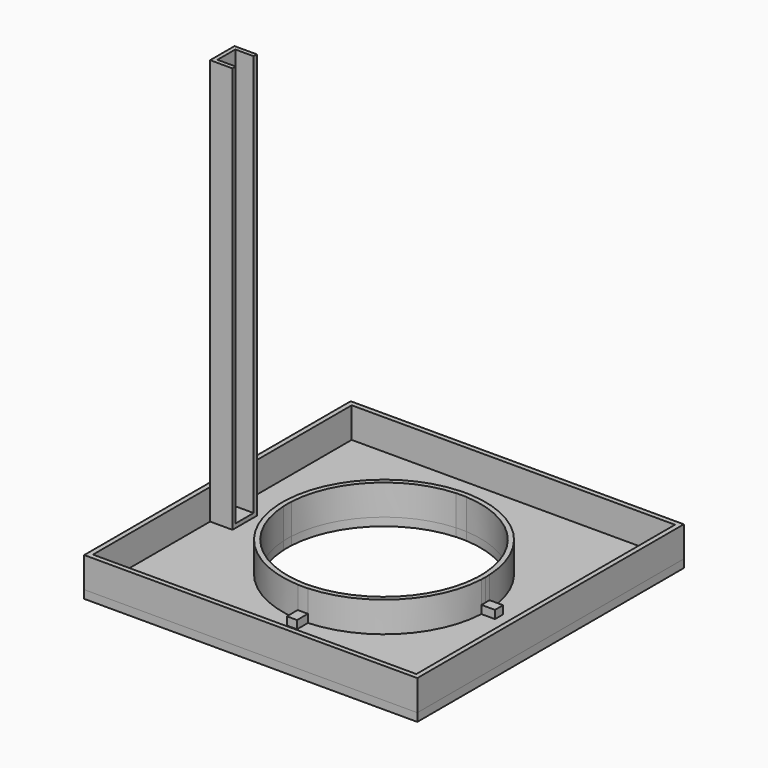
from build123d import *

# Parameters (mm, degrees)
F1_DEPTH = 7.5
F0_W     = 82
F0_H     = 82
F0_R     = 32.8
F0_W_2   = 5.5
F0_H_2   = 7.5
F2_DEPTH = 2
F3_DEPTH = 2
F4_DEPTH = 100
F5_T     = -1


# Not quite as in the source:
# - a feature names something its author has since deleted; it is built from what else it names


with BuildPart() as f1:
    # F0 (on Top) → F1 (new body)
    with BuildSketch(Plane.XY):
        with BuildLine():
            ThreePointArc((-24.9687304443, -1.25), (-17.6776695297, -17.6776695297), (-1.25, -24.9687304443))
            Line((-1.25, -24.9687304443), (-1.25, -23.7671517015))
            ThreePointArc((-1.25, -23.7671517015), (-16.8291413922, -16.8291413922), (-23.7671517015, -1.25))
            Line((-23.7671517015, -1.25), (-24.9687304443, -1.25))
        make_face()
        with BuildLine():
            Line((-1.25, 23.7671517015), (-1.25, 24.9687304443))
            ThreePointArc((-1.25, 24.9687304443), (-17.6776695297, 17.6776695297), (-24.9687304443, 1.25))
            Line((-24.9687304443, 1.25), (-23.7671517015, 1.25))
            ThreePointArc((-23.7671517015, 1.25), (-16.8291413922, 16.8291413922), (-1.25, 23.7671517015))
        make_face()
        with BuildLine():
            Line((23.7671517015, 1.25), (24.9687304443, 1.25))
            ThreePointArc((24.9687304443, 1.25), (17.6776695297, 17.6776695297), (1.25, 24.9687304443))
            Line((1.25, 24.9687304443), (1.25, 23.7671517015))
            ThreePointArc((1.25, 23.7671517015), (16.8291413922, 16.8291413922), (23.7671517015, 1.25))
        make_face()
        with BuildLine():
            ThreePointArc((1.25, -24.9687304443), (17.6776695297, -17.6776695297), (24.9687304443, -1.25))
            Line((24.9687304443, -1.25), (23.7671517015, -1.25))
            ThreePointArc((23.7671517015, -1.25), (16.8291413922, -16.8291413922), (1.25, -23.7671517015))
            Line((1.25, -23.7671517015), (1.25, -24.9687304443))
        make_face()
        with BuildLine():
            Line((1.25, 23.7671517015), (1.25, 24.9687304443))
            ThreePointArc((1.25, 24.9687304443), (0, 25), (-1.25, 24.9687304443))
            Line((-1.25, 24.9687304443), (-1.25, 23.7671517015))
            ThreePointArc((-1.25, 23.7671517015), (0, 23.8), (1.25, 23.7671517015))
        make_face()
        with BuildLine():
            ThreePointArc((-1.25, -24.9687304443), (0, -25), (1.25, -24.9687304443))
            Line((1.25, -24.9687304443), (1.25, -23.7671517015))
            ThreePointArc((1.25, -23.7671517015), (0, -23.8), (-1.25, -23.7671517015))
            Line((-1.25, -23.7671517015), (-1.25, -24.9687304443))
        make_face()
        with BuildLine():
            ThreePointArc((24.9687304443, -1.25), (24.9921813885, -0.6251955264), (25, 0))
            ThreePointArc((25, 0), (24.9921813885, 0.6251955264), (24.9687304443, 1.25))
            Line((24.9687304443, 1.25), (23.7671517015, 1.25))
            ThreePointArc((23.7671517015, 1.25), (23.7917865081, 0.6252157649), (23.8, 0))
            ThreePointArc((23.8, 0), (23.7917865081, -0.6252157649), (23.7671517015, -1.25))
            Line((23.7671517015, -1.25), (24.9687304443, -1.25))
        make_face()
        with BuildLine():
            Line((-23.7671517015, 1.25), (-24.9687304443, 1.25))
            ThreePointArc((-24.9687304443, 1.25), (-25, 0), (-24.9687304443, -1.25))
            Line((-24.9687304443, -1.25), (-23.7671517015, -1.25))
            ThreePointArc((-23.7671517015, -1.25), (-23.8, 0), (-23.7671517015, 1.25))
        make_face()
    extrude(amount=F1_DEPTH)


with BuildPart() as f1b:
    # F0 (on Top) → F1, piece 2 (new body)
    with BuildSketch(Plane.XY):
        Rectangle(F0_W, F0_H)
        Polygon((-39.8, 3.75), (-39.8, 39.8), (39.8, 39.8), (39.8, -39.8), (-39.8, -39.8), (-39.8, -3.75), align=None, mode=Mode.SUBTRACT)
    extrude(amount=F1_DEPTH)


with BuildPart() as f2:
    # F0 (on Top) → F2 (new body)
    with BuildSketch(Plane.XY):
        Rectangle(F0_W, F0_H)
        Polygon((-39.8, 3.75), (-39.8, 39.8), (39.8, 39.8), (39.8, -39.8), (-39.8, -39.8), (-39.8, -3.75), align=None, mode=Mode.SUBTRACT)
        Polygon((39.8, 39.8), (-39.8, 39.8), (-39.8, 3.75), (-34.3, 3.75), (-34.3, -3.75), (-39.8, -3.75), (-39.8, -39.8), (39.8, -39.8), align=None)
        Circle(F0_R, mode=Mode.SUBTRACT)
        Circle(F0_R)
        with BuildLine():
            ThreePointArc((1.25, 24.9687304443), (17.6776695297, 17.6776695297), (24.9687304443, 1.25))
            Line((24.9687304443, 1.25), (28.325, 1.25))
            Line((28.325, 1.25), (28.325, -1.25))
            Line((28.325, -1.25), (24.9687304443, -1.25))
            ThreePointArc((24.9687304443, -1.25), (17.6776695297, -17.6776695297), (1.25, -24.9687304443))
            Line((1.25, -24.9687304443), (1.25, -28.325))
            Line((1.25, -28.325), (-1.25, -28.325))
            Line((-1.25, -28.325), (-1.25, -24.9687304443))
            ThreePointArc((-1.25, -24.9687304443), (-17.6776695297, -17.6776695297), (-24.9687304443, -1.25))
            Line((-24.9687304443, -1.25), (-28.325, -1.25))
            Line((-28.325, -1.25), (-28.325, 1.25))
            Line((-28.325, 1.25), (-24.9687304443, 1.25))
            ThreePointArc((-24.9687304443, 1.25), (-17.6776695297, 17.6776695297), (-1.25, 24.9687304443))
            Line((-1.25, 24.9687304443), (-1.25, 28.325))
            Line((-1.25, 28.325), (1.25, 28.325))
            Line((1.25, 28.325), (1.25, 24.9687304443))
        make_face(mode=Mode.SUBTRACT)
        with BuildLine():
            Line((23.7671517015, 1.25), (24.9687304443, 1.25))
            ThreePointArc((24.9687304443, 1.25), (17.6776695297, 17.6776695297), (1.25, 24.9687304443))
            Line((1.25, 24.9687304443), (1.25, 23.7671517015))
            ThreePointArc((1.25, 23.7671517015), (16.8291413922, 16.8291413922), (23.7671517015, 1.25))
        make_face()
        with BuildLine():
            Line((-1.25, 23.7671517015), (-1.25, 24.9687304443))
            ThreePointArc((-1.25, 24.9687304443), (-17.6776695297, 17.6776695297), (-24.9687304443, 1.25))
            Line((-24.9687304443, 1.25), (-23.7671517015, 1.25))
            ThreePointArc((-23.7671517015, 1.25), (-16.8291413922, 16.8291413922), (-1.25, 23.7671517015))
        make_face()
        with BuildLine():
            ThreePointArc((-24.9687304443, -1.25), (-17.6776695297, -17.6776695297), (-1.25, -24.9687304443))
            Line((-1.25, -24.9687304443), (-1.25, -23.7671517015))
            ThreePointArc((-1.25, -23.7671517015), (-16.8291413922, -16.8291413922), (-23.7671517015, -1.25))
            Line((-23.7671517015, -1.25), (-24.9687304443, -1.25))
        make_face()
        with BuildLine():
            ThreePointArc((1.25, -24.9687304443), (17.6776695297, -17.6776695297), (24.9687304443, -1.25))
            Line((24.9687304443, -1.25), (23.7671517015, -1.25))
            ThreePointArc((23.7671517015, -1.25), (16.8291413922, -16.8291413922), (1.25, -23.7671517015))
            Line((1.25, -23.7671517015), (1.25, -24.9687304443))
        make_face()
        with Locations((-37.05, 0)):
            Rectangle(F0_W_2, F0_H_2)
        with BuildLine():
            ThreePointArc((-24.9687304443, -1.25), (-25, 0), (-24.9687304443, 1.25))
            Line((-24.9687304443, 1.25), (-28.325, 1.25))
            Line((-28.325, 1.25), (-28.325, -1.25))
            Line((-28.325, -1.25), (-24.9687304443, -1.25))
        make_face()
        with BuildLine():
            Line((1.25, -28.325), (1.25, -24.9687304443))
            ThreePointArc((1.25, -24.9687304443), (0, -25), (-1.25, -24.9687304443))
            Line((-1.25, -24.9687304443), (-1.25, -28.325))
            Line((-1.25, -28.325), (1.25, -28.325))
        make_face()
        with BuildLine():
            ThreePointArc((-1.25, 24.9687304443), (0, 25), (1.25, 24.9687304443))
            Line((1.25, 24.9687304443), (1.25, 28.325))
            Line((1.25, 28.325), (-1.25, 28.325))
            Line((-1.25, 28.325), (-1.25, 24.9687304443))
        make_face()
        with BuildLine():
            ThreePointArc((24.9687304443, 1.25), (24.9921813885, 0.6251955264), (25, 0))
            ThreePointArc((25, 0), (24.9921813885, -0.6251955264), (24.9687304443, -1.25))
            Line((24.9687304443, -1.25), (28.325, -1.25))
            Line((28.325, -1.25), (28.325, 1.25))
            Line((28.325, 1.25), (24.9687304443, 1.25))
        make_face()
        with BuildLine():
            Line((1.25, 23.7671517015), (1.25, 24.9687304443))
            ThreePointArc((1.25, 24.9687304443), (0, 25), (-1.25, 24.9687304443))
            Line((-1.25, 24.9687304443), (-1.25, 23.7671517015))
            ThreePointArc((-1.25, 23.7671517015), (0, 23.8), (1.25, 23.7671517015))
        make_face()
        with BuildLine():
            Line((-23.7671517015, 1.25), (-24.9687304443, 1.25))
            ThreePointArc((-24.9687304443, 1.25), (-25, 0), (-24.9687304443, -1.25))
            Line((-24.9687304443, -1.25), (-23.7671517015, -1.25))
            ThreePointArc((-23.7671517015, -1.25), (-23.8, 0), (-23.7671517015, 1.25))
        make_face()
        with BuildLine():
            ThreePointArc((-1.25, -24.9687304443), (0, -25), (1.25, -24.9687304443))
            Line((1.25, -24.9687304443), (1.25, -23.7671517015))
            ThreePointArc((1.25, -23.7671517015), (0, -23.8), (-1.25, -23.7671517015))
            Line((-1.25, -23.7671517015), (-1.25, -24.9687304443))
        make_face()
        with BuildLine():
            ThreePointArc((24.9687304443, -1.25), (24.9921813885, -0.6251955264), (25, 0))
            ThreePointArc((25, 0), (24.9921813885, 0.6251955264), (24.9687304443, 1.25))
            Line((24.9687304443, 1.25), (23.7671517015, 1.25))
            ThreePointArc((23.7671517015, 1.25), (23.7917865081, 0.6252157649), (23.8, 0))
            ThreePointArc((23.8, 0), (23.7917865081, -0.6252157649), (23.7671517015, -1.25))
            Line((23.7671517015, -1.25), (24.9687304443, -1.25))
        make_face()
    extrude(amount=-F2_DEPTH)


with BuildPart() as f3:
    # F0 (on Top) → F3 (new body)
    with BuildSketch(Plane.XY):
        with BuildLine():
            ThreePointArc((-24.9687304443, -1.25), (-25, 0), (-24.9687304443, 1.25))
            Line((-24.9687304443, 1.25), (-28.325, 1.25))
            Line((-28.325, 1.25), (-28.325, -1.25))
            Line((-28.325, -1.25), (-24.9687304443, -1.25))
        make_face()
    extrude(amount=F3_DEPTH)


with BuildPart() as f3b:
    # F0 (on Top) → F3, piece 2 (new body)
    with BuildSketch(Plane.XY):
        with BuildLine():
            ThreePointArc((-1.25, 24.9687304443), (0, 25), (1.25, 24.9687304443))
            Line((1.25, 24.9687304443), (1.25, 28.325))
            Line((1.25, 28.325), (-1.25, 28.325))
            Line((-1.25, 28.325), (-1.25, 24.9687304443))
        make_face()
    extrude(amount=F3_DEPTH)


with BuildPart() as f3c:
    # F0 (on Top) → F3, piece 3 (new body)
    with BuildSketch(Plane.XY):
        with BuildLine():
            ThreePointArc((24.9687304443, 1.25), (24.9921813885, 0.6251955264), (25, 0))
            ThreePointArc((25, 0), (24.9921813885, -0.6251955264), (24.9687304443, -1.25))
            Line((24.9687304443, -1.25), (28.325, -1.25))
            Line((28.325, -1.25), (28.325, 1.25))
            Line((28.325, 1.25), (24.9687304443, 1.25))
        make_face()
    extrude(amount=F3_DEPTH)


with BuildPart() as f3d:
    # F0 (on Top) → F3, piece 4 (new body)
    with BuildSketch(Plane.XY):
        with BuildLine():
            Line((1.25, -28.325), (1.25, -24.9687304443))
            ThreePointArc((1.25, -24.9687304443), (0, -25), (-1.25, -24.9687304443))
            Line((-1.25, -24.9687304443), (-1.25, -28.325))
            Line((-1.25, -28.325), (1.25, -28.325))
        make_face()
    extrude(amount=F3_DEPTH)


with BuildPart() as f4:
    # F0 (on Top) → F4 (new body)
    with BuildSketch(Plane.XY):
        with Locations((-37.05, 0)):
            Rectangle(F0_W_2, F0_H_2)
    extrude(amount=F4_DEPTH)

    # F5
    f5_openings = [f4.faces().sort_by_distance(p)[0] for p in [
        (-37.05, 0, 100),
        (-34.3, 0, 50),
    ]]
    offset(amount=F5_T, openings=f5_openings)


solid = Compound([f1.part, f1b.part, f2.part, f3.part, f3b.part, f3c.part, f3d.part, f4.part])
